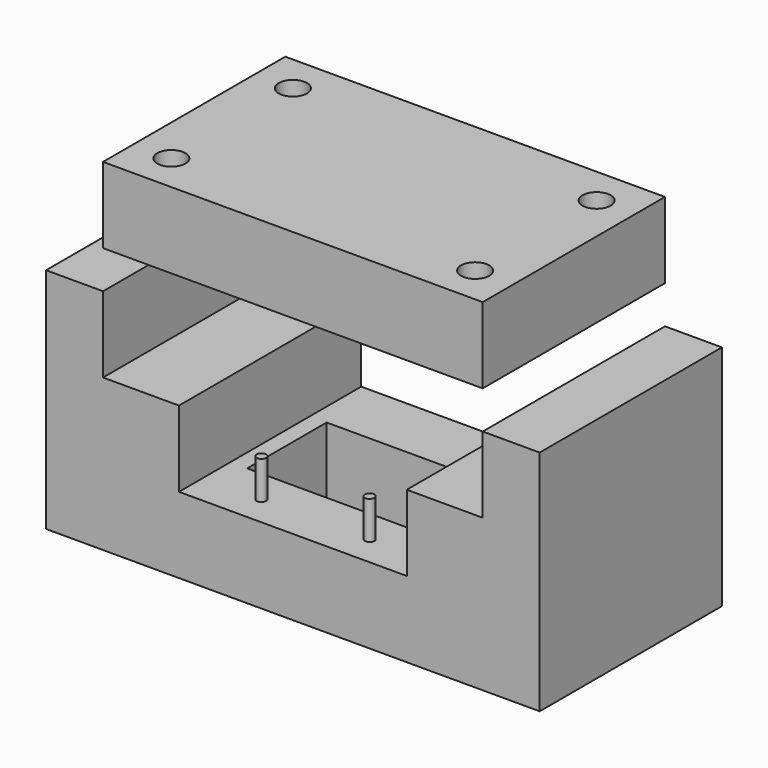
from build123d import *

# Parameters (mm, degrees)
F6_W      = 76.2
F6_H      = 50.8
F7_DEPTH  = 152.4
F0_W      = 129.9560666084
F0_H      = 66.4875675201
F1_DEPTH  = 50.801
F9_DEPTH  = 152.4
F2_R      = 3.175
F3_DEPTH  = 25.4
F4_R      = 9.4371110392
F10_DEPTH = 228.601


with BuildPart() as f7:
    # F6 (on Front) → F7 (new body)
    with BuildSketch(Plane.XZ):
        Polygon((0, 152.4), (0, 0), (38.1, 0), (38.1, 101.6), (38.1, 152.4), align=None)
        with Locations((127, 25.4)):
            Rectangle(F6_W, F6_H)
        Polygon((38.1, 101.6), (38.1, 0), (88.9, 0), (88.9, 50.8), (88.9, 101.6), align=None)
        with Locations((203.2, 25.4)):
            Rectangle(F6_W, F6_H)
        Polygon((241.3, 50.8), (241.3, 0), (292.1, 0), (292.1, 101.6), (241.3, 101.6), align=None)
        Polygon((292.1, 101.6), (292.1, 0), (330.2, 0), (330.2, 152.4), (292.1, 152.4), align=None)
    extrude(amount=-F7_DEPTH)

    # F0 (on face) → F1 (cut, through all)
    with BuildSketch(Plane.XY.offset(50.8)):
        with Locations((165.1, 76.2)):
            Rectangle(F0_W, F0_H)
    extrude(amount=-F1_DEPTH, mode=Mode.SUBTRACT)

    # F2 (on face) → F3 (join)
    with BuildSketch(Plane.XY.offset(50.8)):
        with Locations((127.7533173561, 20.32)):
            Circle(F2_R)
        with Locations((200.1881897449, 20.32)):
            Circle(F2_R)
    extrude(amount=F3_DEPTH)


with BuildPart() as f9:
    # F8 (on Front) → F9 (new body)
    with BuildSketch(Plane.XZ):
        Polygon((38.1, 228.6), (38.1, 177.8), (139.7, 177.8), (190.5, 177.8), (292.1, 177.8), (292.1, 228.6), align=None)
    extrude(amount=-F9_DEPTH)

    # F4 (on face) → F10 (cut, through all)
    with BuildSketch(Plane.XY.offset(228.6)):
        with Locations((63.5, 25.4)):
            Circle(F4_R)
        with Locations((63.5, 127)):
            Circle(F4_R)
        with Locations((266.7, 25.4)):
            Circle(F4_R)
        with Locations((266.7, 127)):
            Circle(F4_R)
    extrude(amount=-F10_DEPTH, mode=Mode.SUBTRACT)


solid = Compound([f7.part, f9.part])
